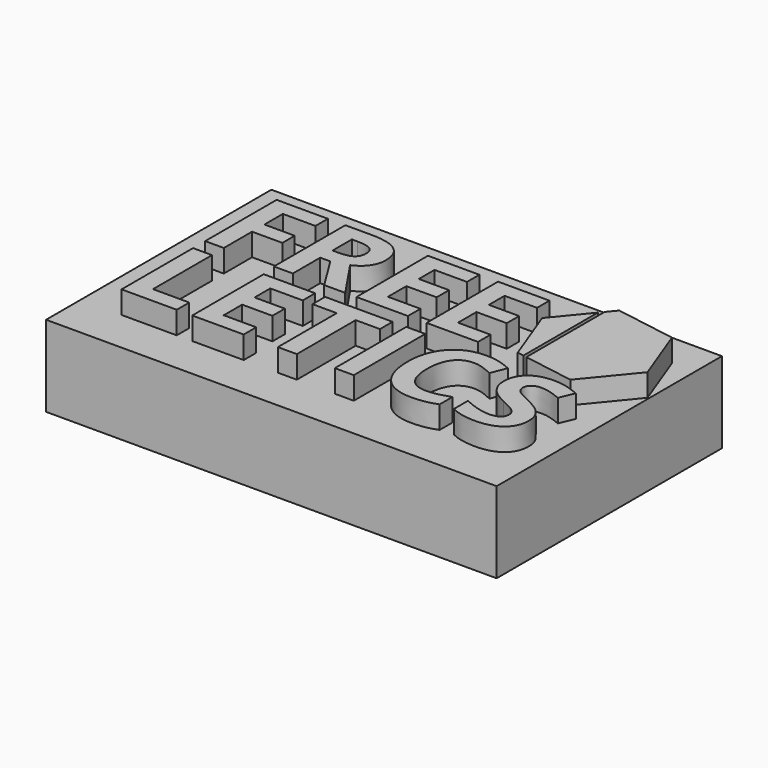
from build123d import *

# Parameters (mm, degrees)
F0_R         = 11.6
F0_R_2       = 9.6
F1_DEPTH     = 5.2
F2_R         = 11.6
F2_R_2       = 9.6
F3_DEPTH     = 2
F4_W         = 40
F4_H         = 25
F4_R         = 11.6
F5_DEPTH     = 7.2
F6_TEXT_SIZE = 11.1111111111
F7_DEPTH     = 2
F9_DEPTH     = 2
F10_W        = 0.3039054573
F10_H        = 10.1175568998
F11_DEPTH    = 2


# Not quite as in the source:
# - Text() gives the source's letters only with a copy of the font that has no kerning and outlines rounded to 1/6400 em; it was checked with that copy


with BuildPart() as f1:
    # F0 (on Top) → F1 (new body)
    with BuildSketch(Plane.XY):
        Circle(F0_R)
        Circle(F0_R_2, mode=Mode.SUBTRACT)
    extrude(amount=F1_DEPTH)

    # F2 (on face) → F3 (join)
    with BuildSketch(Plane.XY.offset(5.2)):
        Circle(F2_R)
        Circle(F2_R_2, mode=Mode.SUBTRACT)
        Circle(F2_R_2)
    extrude(amount=F3_DEPTH)

    # F4 (on face) → F5 (join)
    with BuildSketch(Plane.XY.offset(7.2)):
        Rectangle(F4_W, F4_H)
        Circle(F4_R, mode=Mode.SUBTRACT)
    extrude(amount=-F5_DEPTH)

    # F6 (on face) → F7 (join)
    with BuildSketch(Plane.XY.offset(7.2)):
        with Locations((-17.3616698538, 0.6079855682)):
            Text('FREE', F6_TEXT_SIZE, font='Open Sans', font_style=FontStyle.BOLD, text_align=(TextAlign.LEFT, TextAlign.BOTTOM))
        with Locations((-17.3616698538, -8.6712793739)):
            Text('LETICS', F6_TEXT_SIZE, font='Open Sans', font_style=FontStyle.BOLD, text_align=(TextAlign.LEFT, TextAlign.BOTTOM))
    extrude(amount=F7_DEPTH)

    # F8 (on face) → F9 (join)
    with BuildSketch(Plane.XY.offset(7.2)):
        Polygon((12.5652893801, 10.405062506), (9.0951032614, 6.1840116605), (11.0155474649, 1.0682169031), (16.4061777871, 0.1734729912), (19.8763639057, 4.3945238367), (17.9559197023, 9.510318594), align=None)
    extrude(amount=F9_DEPTH)

    # F10 (on face) → F11 (cut)
    with BuildSketch(Plane.XY.offset(9.2)):
        with Locations((11.7514925078, 5.0587784499)):
            Rectangle(F10_W, F10_H)
    extrude(amount=-F11_DEPTH, mode=Mode.SUBTRACT)


solid = f1.part
